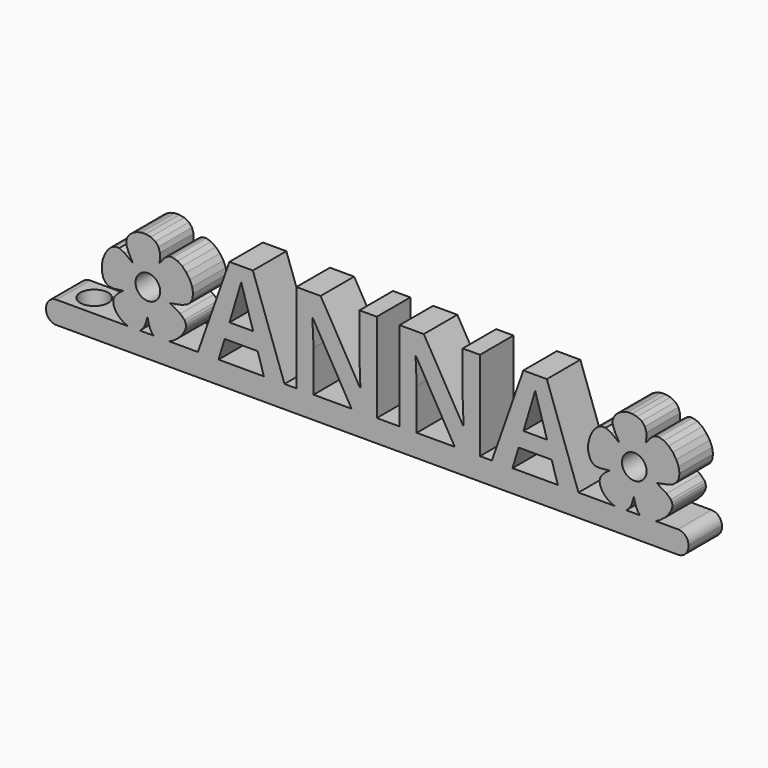
from build123d import *

# Parameters (mm, degrees)
F0_R         = 1.7660260944
F0_TEXT_SIZE = 18.1803425047
F1_DEPTH     = 3
F2_W         = 84.5
F2_H         = 6
F3_DEPTH     = 0.2
F4_DEPTH     = 3
F5_W         = 6
F5_H         = 3.2
F6_DEPTH     = 7.5
F7_R         = 1.5
F8_R         = 2
F9_DEPTH     = 4
F10_R        = 1.5


# Not quite as in the source:
# - Text() gives the source's letters only with a copy of the font that has no kerning and outlines rounded to 1/6400 em; it was checked with that copy


with BuildPart() as f1:
    # F0 (on Front) → F1 (new body, symmetric)
    with BuildSketch(Plane.XZ):
        Polygon((-9.8962181259, -0.0299609487), (-9.3093152472, 0.0995427735), (-8.5310452338, 0.4643787281), (-7.7886221935, 1.0156229815), (-7.1753136859, 1.6703047867), (-6.7844076966, 2.345448762), (-6.6844409889, 2.697736103), (-6.6652413988, 3.0240118702), (-6.7312263226, 3.3305926174), (-6.8868132072, 3.6238062576), (-7.4844896445, 4.1953846804), (-8.4936258745, 4.789299945), (-8.9274018823, 5.0567831788), (-8.4181052429, 5.1580766137), (-7.3131137554, 5.3695361907), (-6.5480905692, 5.6521941874), (-6.0523445823, 6.043851435), (-5.7552051187, 6.5823041299), (-5.6420905942, 7.3346827833), (-5.7751165223, 8.1369112107), (-6.1089634595, 8.9328581362), (-6.5983028952, 9.6663968681), (-7.1978267956, 10.281407439), (-7.8622157172, 10.7217585729), (-8.546147975, 10.9313258196), (-8.8812811082, 10.9320270148), (-9.2043064176, 10.8539824368), (-9.6469000392, 10.5612860557), (-10.1400767255, 9.9810366231), (-10.4508130024, 9.5801644376), (-10.4068223535, 10.0271686751), (-10.3916193646, 10.9311557532), (-10.598433195, 11.6324207168), (-11.0363252865, 12.1480644274), (-11.7143548393, 12.4951945719), (-12.3982545289, 12.6383143795), (-13.0712303381, 12.6247535348), (-13.7032208938, 12.4733707309), (-14.2641853, 12.2030313855), (-14.7240621838, 11.8325941916), (-15.0528129411, 11.3809291004), (-15.2203761991, 10.8668948051), (-15.1967042361, 10.3093544817), (-14.8286469794, 9.4077545862), (-14.3529716358, 8.5454741101), (-14.2906102139, 8.4004774316), (-14.4811582303, 8.5293860258), (-15.3946726039, 9.2300894295), (-16.21802192, 9.6332437342), (-16.8030362894, 9.634121823), (-17.3568401554, 9.3699870508), (-17.8525159958, 8.8932532172), (-18.2631576982, 8.2563454299), (-18.5618432066, 7.5116797807), (-18.7216618753, 6.7116836696), (-18.7156984739, 5.9087754295), (-18.5170445979, 5.1553756349), (-18.2008868091, 4.6439944488), (-17.7512302174, 4.3560670179), (-17.1086136552, 4.2712956407), (-16.2135760559, 4.3694053341), (-15.7044514474, 4.4302814773), (-15.6696932647, 4.4000047008), (-15.7790195709, 4.3290260096), (-16.1651405309, 4.0708069691), (-16.5523139664, 3.7127982689), (-16.8671052824, 3.3322639471), (-17.0360798838, 3.0064680418), (-17.0831036318, 2.6043628391), (-17.0239245605, 2.1921008316), (-16.867618816, 1.7819255621), (-16.6232807801, 1.3860941234), (-16.3000002503, 1.0168545414), (-15.9068693162, 0.6864593752), (-15.4529754831, 0.4071521172), (-14.9474063577, 0.1911989779), (-14.4397479673, 0.0570083052), (-13.9840845603, 0.0188926715), (-13.5797273957, 0.0772799851), (-13.2259605822, 0.2326232662), (-12.9220907946, 0.485341356), (-12.6674066752, 0.8358849825), (-12.4612081239, 1.2846821047), (-12.3027905578, 1.8321743328), (-12.1879723822, 2.2557758958), (-12.1309056827, 2.0998483864), (-12.0112204133, 1.5291342486), (-11.8237778137, 0.9902805659), (-11.5954117235, 0.5466869075), (-11.3529559319, 0.2617414835), (-10.9521058183, 0.053843468), (-10.4551700276, -0.0442881949), align=None)
        with Locations((-12.1185852993, 6.0541479067)):
            Circle(F0_R, mode=Mode.SUBTRACT)
        Polygon((59.526901838, 9.9810366231), (59.2161655612, 9.5801644376), (59.26015621, 10.0271686751), (59.2753591989, 10.9311557532), (59.0685453685, 11.6324207168), (58.6306532771, 12.1480644274), (57.9526237243, 12.4951945719), (57.2687240346, 12.6383143795), (56.5957482255, 12.6247535348), (55.9637576698, 12.4733707309), (55.4027932636, 12.2030313855), (54.9429163798, 11.8325941916), (54.6141656224, 11.3809291004), (54.4466023644, 10.8668948051), (54.4702743274, 10.3093544817), (54.8383315841, 9.4077545862), (55.3140069277, 8.5454741101), (55.3763683496, 8.4004774316), (55.1858203332, 8.5293860258), (54.2723059597, 9.2300894295), (53.4489566436, 9.6332437342), (52.8639422742, 9.634121823), (52.3101384081, 9.3699870508), (51.8144625677, 8.8932532172), (51.4038208654, 8.2563454299), (51.1051353569, 7.5116797807), (50.9453166883, 6.7116836696), (50.9512800897, 5.9087754295), (51.1499339657, 5.1553756349), (51.4660917545, 4.6439944488), (51.9157483462, 4.3560670179), (52.5583649084, 4.2712956407), (53.4534025077, 4.3694053341), (53.9625271162, 4.4302814773), (53.9972852989, 4.4000047008), (53.8879589927, 4.3290260096), (53.5018380327, 4.0708069691), (53.1146645972, 3.7127982689), (52.7998732812, 3.3322639471), (52.6308986797, 3.0064680418), (52.5838749317, 2.6043628391), (52.6430540031, 2.1921008316), (52.7993597475, 1.7819255621), (53.0436977834, 1.3860941234), (53.3669783132, 1.0168545414), (53.7601092474, 0.6864593752), (54.2140030805, 0.4071521172), (54.7195722058, 0.1911989779), (55.2272305962, 0.0570083052), (55.6828940033, 0.0188926715), (56.0872511678, 0.0772799851), (56.4410179814, 0.2326232662), (56.7448877689, 0.485341356), (56.9995718883, 0.8358849825), (57.2057704397, 1.2846821047), (57.3641880058, 1.8321743328), (57.4790061813, 2.2557758958), (57.5360728808, 2.0998483864), (57.6557581502, 1.5291342486), (57.8432007498, 0.9902805659), (58.07156684, 0.5466869075), (58.3140226317, 0.2617414835), (58.7148727453, 0.053843468), (59.211808536, -0.0442881949), (59.7707604376, -0.0299609487), (60.3576633164, 0.0995427735), (61.1359333298, 0.4643787281), (61.87835637, 1.0156229815), (62.4916648777, 1.6703047867), (62.8825708669, 2.345448762), (62.9825375747, 2.697736103), (63.0017371647, 3.0240118702), (62.9357522409, 3.3305926174), (62.7801653564, 3.6238062576), (62.1824889191, 4.1953846804), (61.173352689, 4.789299945), (60.7395766813, 5.0567831788), (61.2488733207, 5.1580766137), (62.3538648082, 5.3695361907), (63.1188879943, 5.6521941874), (63.6146339812, 6.043851435), (63.9117734448, 6.5823041299), (64.0248879693, 7.3346827833), (63.8918620412, 8.1369112107), (63.558015104, 8.9328581362), (63.0686756684, 9.6663968681), (62.4691517679, 10.281407439), (61.8047628464, 10.7217585729), (61.1208305885, 10.9313258196), (60.7856974553, 10.9320270148), (60.462672146, 10.8539824368), (60.0200785243, 10.5612860557), align=None)
        with Locations((57.5483932642, 6.0541479067)):
            Circle(F0_R, mode=Mode.SUBTRACT)
        with Locations((-5.0278548819, 0)):
            Text('ANNA', F0_TEXT_SIZE, font='Open Sans', font_style=FontStyle.BOLD, text_align=(TextAlign.LEFT, TextAlign.BOTTOM))
    extrude(amount=F1_DEPTH, both=True)



with BuildPart() as f3:
    # F2 (on Top) → F3 (new body)
    with BuildSketch(Plane.XY):
        with Locations((23.05, 0)):
            Rectangle(F2_W, F2_H)
    extrude(amount=F3_DEPTH)


with BuildPart() as f4:
    # F4 (new): a face of the model
    f4_faces = [f3.part.faces().sort_by_distance(p)[0] for p in [
        (23.05, 0, 0),
    ]]
    extrude(f4_faces, amount=F4_DEPTH)


with BuildPart() as f1_1:
    add(f1.part)

    add(f3.part)  # F6 merges F3

    add(f4.part)  # F6 merges F4
    # F5 (on face) → F6 (join)
    with BuildSketch(Plane(origin=(-19.2, 0, 0), x_dir=(0, -1, 0), z_dir=(-1, 0, 0))):
        with Locations((0, -1.4)):
            Rectangle(F5_W, F5_H)
    extrude(amount=F6_DEPTH)

    # F7
    f7_edges = [f1_1.edges().sort_by_distance(p)[0] for p in [
        (-26.7, 0, -3),
        (-26.7, 0, 0.2),
        (65.3, 0, -3),
    ]]
    fillet(f7_edges, radius=F7_R)

    # F8 (on face) → F9 (cut)
    with BuildSketch(Plane.XY.offset(0.2)):
        with Locations((-22.2, 0)):
            Circle(F8_R)
    extrude(amount=-F9_DEPTH, mode=Mode.SUBTRACT)

    # F10
    f10_edges = [f1_1.edges().sort_by_distance(p)[0] for p in [
        (65.3, 0, 0.2),
    ]]
    fillet(f10_edges, radius=F10_R)


solid = f1_1.part
